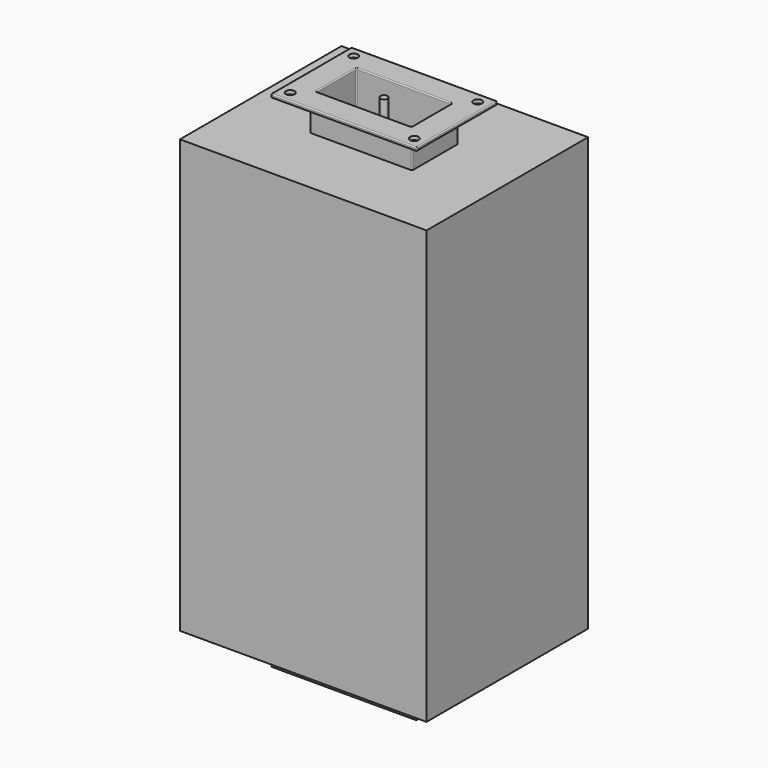
from build123d import *

# Parameters (mm, degrees)
F0_W     = 142
F0_H     = 80
F1_DEPTH = 350
F2_W     = 202
F2_H     = 140
F2_R     = 6
F2_W_2   = 131.9999952316
F2_H_2   = 69.9999952316
F3_DEPTH = 5
F2_R_2   = 5
F5_DEPTH = 700
F6_R     = 1.5
F7_W     = 342
F7_H     = 280
F8_DEPTH = 300


with BuildPart() as f1:
    # F0 (on Top) → F1 (new body)
    with BuildSketch(Plane.XY):
        Rectangle(F0_W, F0_H)
    extrude(amount=F1_DEPTH)

    # F2 (on Top) → F3 (join)
    with BuildSketch(Plane.XY):
        Rectangle(F2_W, F2_H)
        with Locations((-86, -55)):
            Circle(F2_R, mode=Mode.SUBTRACT)
        with Locations((86, -55)):
            Circle(F2_R, mode=Mode.SUBTRACT)
        with Locations((-86, 55)):
            Circle(F2_R, mode=Mode.SUBTRACT)
        Rectangle(F2_W_2, F2_H_2, mode=Mode.SUBTRACT)
        with Locations((86, 55)):
            Circle(F2_R, mode=Mode.SUBTRACT)
    extrude(amount=F3_DEPTH)

    # F4: union 

    # F2 (on Top) → F5 (cut)
    with BuildSketch(Plane.XY):
        Rectangle(F2_W_2, F2_H_2)
        Circle(F2_R_2, mode=Mode.SUBTRACT)
    extrude(amount=F5_DEPTH, mode=Mode.SUBTRACT)

    # F6
    f6_edges = [f1.edges().sort_by_distance(p)[0] for p in [
        (0, 40, 5),
        (101, 0, 5),
        (0, 70, 0),
        (65.999998, -34.999998, 175),
        (-101, 0, 0),
        (0, -70, 5),
        (101, 70, 2.5),
        (0, 70, 5),
        (71, -40, 177.5),
        (65.999998, 34.999998, 175),
        (71, 0, 5),
        (101, -70, 2.5),
        (0, -70, 0),
        (-101, 0, 5),
        (-71, 40, 177.5),
        (101, 0, 0),
        (71, 40, 177.5),
        (-65.999998, 34.999998, 175),
        (-65.999998, -34.999998, 175),
        (0, 34.999998, 0),
        (0, -34.999998, 0),
        (0, -40, 5),
        (-101, 70, 2.5),
        (-101, -70, 2.5),
        (-71, 0, 5),
        (-71, -40, 177.5),
        (65.999998, 0, 0),
        (-65.999998, 0, 0),
    ]]
    fillet(f6_edges, radius=F6_R)

    # F7 (on face) → F8 (join)
    with BuildSketch(Plane.XY.offset(350)):
        Rectangle(F7_W, F7_H)
    extrude(amount=-F8_DEPTH)

    # F9: F1 across face


with BuildPart() as f1_1:
    add(f1.part)
    add(f1.part.mirror(Plane.XY.offset(350)))


solid = f1_1.part
